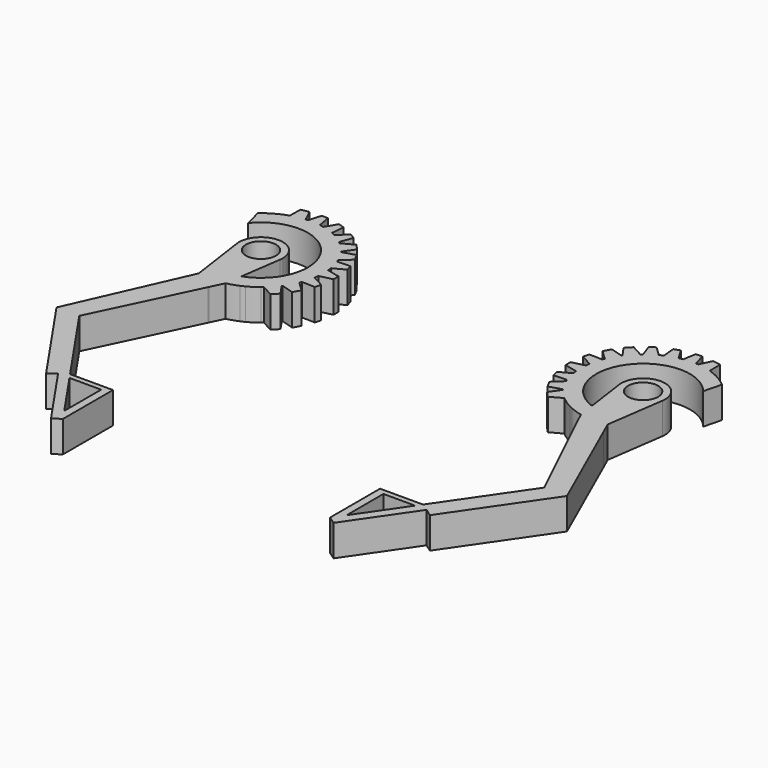
from build123d import *

# Parameters (mm, degrees)
F0_R     = 2.4
F1_DEPTH = 5
F2_DEPTH = 5


# Not quite as in the source:
# - a feature names something its author has since deleted; it is built from what else it names


with BuildPart() as f1:
    # F0 (on Top) → F1 (new body)
    with BuildSketch(Plane.XY):
        with BuildLine():
            Line((-28.0220931123, -7.0605402827), (-28.4076857165, -9.7674623873))
            ThreePointArc((-28.4076857165, -9.7674623873), (-27.4606084204, -9.510274656), (-26.5433011896, -9.1614933807))
            ThreePointArc((-26.5433011896, -9.1614933807), (-26.2465613416, -9.0258528435), (-25.9544044087, -8.8806040249))
            ThreePointArc((-25.9544044087, -8.8806040249), (-25.1052819595, -8.3867056795), (-24.3087141549, -7.811880278))
            ThreePointArc((-24.3087141549, -7.811880278), (-24.1632529957, -7.6933801849), (-24.0200406381, -7.572171928))
            ThreePointArc((-24.0200406381, -7.572171928), (-23.2137191877, -6.7937062036), (-22.4995744015, -5.9299004442))
            ThreePointArc((-22.4995744015, -5.9299004442), (-22.4615023659, -5.8778525229), (-22.4237667572, -5.8255601731))
            ThreePointArc((-22.4237667572, -5.8255601731), (-21.8229215363, -4.8794374612), (-21.3317236675, -3.8720210532))
            ThreePointArc((-21.3317236675, -3.8720210532), (-21.2607028173, -3.698362596), (-21.1929525017, -3.5234022701))
            ThreePointArc((-21.1929525017, -3.5234022701), (-20.8924140467, -2.588190451), (-20.685082074, -1.6280040303))
            ThreePointArc((-20.685082074, -1.6280040303), (-20.6372236959, -1.3052619222), (-20.5999195351, -0.981130325))
            ThreePointArc((-20.5999195351, -0.981130325), (-20.5516723096, 0), (-20.5999195351, 0.981130325))
            ThreePointArc((-20.5999195351, 0.981130325), (-20.6372236959, 1.3052619222), (-20.685082074, 1.6280040303))
            ThreePointArc((-20.685082074, 1.6280040303), (-20.8924140467, 2.588190451), (-21.1929525017, 3.5234022701))
            ThreePointArc((-21.1929525017, 3.5234022701), (-21.2607028173, 3.698362596), (-21.3317236675, 3.8720210532))
            ThreePointArc((-21.3317236675, 3.8720210532), (-21.8229215363, 4.8794374612), (-22.4237667572, 5.8255601731))
            ThreePointArc((-22.4237667572, 5.8255601731), (-22.4615023659, 5.8778525229), (-22.4995744015, 5.9299004442))
            ThreePointArc((-22.4995744015, 5.9299004442), (-23.2137191877, 6.7937062036), (-24.0200406381, 7.572171928))
            ThreePointArc((-24.0200406381, 7.572171928), (-24.1632529957, 7.6933801849), (-24.3087141549, 7.811880278))
            ThreePointArc((-24.3087141549, 7.811880278), (-25.1052819595, 8.3867056795), (-25.9544044087, 8.8806040249))
            ThreePointArc((-25.9544044087, 8.8806040249), (-26.2465613416, 9.0258528435), (-26.5433011896, 9.1614933807))
            ThreePointArc((-26.5433011896, 9.1614933807), (-27.4615023659, 9.510565163), (-28.4095219674, 9.7678652689))
            ThreePointArc((-28.4095219674, 9.7678652689), (-28.7293170547, 9.8325490756), (-29.0510520919, 9.8867658495))
            ThreePointArc((-29.0510520919, 9.8867658495), (-30.0283127472, 9.9862953475), (-31.0106235319, 9.989462637))
            ThreePointArc((-31.0106235319, 9.989462637), (-31.1979566888, 9.979093972), (-31.3850623458, 9.965212544))
            ThreePointArc((-31.3850623458, 9.965212544), (-32.4949607744, 9.8093644006), (-33.580448329, 9.5302946347))
            ThreePointArc((-33.580448329, 9.5302946347), (-33.6418422534, 9.510565163), (-33.7031076741, 9.4904401976))
            ThreePointArc((-33.7031076741, 9.4904401976), (-34.7453186457, 9.0781788046), (-35.7348505768, 8.5518806734))
            ThreePointArc((-35.7348505768, 8.5518806734), (-35.8943815316, 8.4531330387), (-36.0520317876, 8.3514097979))
            ThreePointArc((-36.0520317876, 8.3514097979), (-36.5923235865, 7.9693495438), (-37.1061642634, 7.5523926823))
            Line((-37.1061642634, 7.5523926823), (-36.3837682078, 4.7155760448))
            ThreePointArc((-36.3837682078, 4.7155760448), (-24.4364549725, 4.3421327617), (-28.0220931123, -7.0605402827))
        make_face()
        with BuildLine():
            ThreePointArc((-34.0166942863, -0.4935815043), (-30.5516723066, -3.5), (-27.0866503321, -0.4935814983))
            ThreePointArc((-27.0866503321, -0.4935814983), (-27.0604277664, -0.247409659), (-27.0516723096, 0))
            ThreePointArc((-27.0516723096, 0), (-30.7990819717, 3.491244543), (-34.0166942863, -0.4935815043))
        make_face()
        with Locations((-30.5516723096, 0)):
            Circle(F0_R, mode=Mode.SUBTRACT)
        with BuildLine():
            Line((-28.4086043831, -9.7693792448), (-28.4076857165, -9.7674623873))
            Line((-28.4076857165, -9.7674623873), (-28.0220931123, -7.0605402827))
            Line((-28.0220931123, -7.0605402827), (-27.0866503321, -0.4935814983))
            ThreePointArc((-27.0866503321, -0.4935814983), (-30.5516723066, -3.5), (-34.0166942863, -0.4935815043))
            Line((-34.0166942863, -0.4935815043), (-32.6956589028, -9.7674623873))
            Line((-32.6956589028, -9.7674623873), (-33.5248075263, -11.635811156))
            Line((-33.5248075263, -11.635811156), (-40.8083886817, -28.0481520771))
            Line((-40.8083886817, -28.0481520771), (-30.6916443131, -42.7764088872))
            Line((-30.6916443131, -42.7764088872), (-29.4552314726, -41.9271249018))
            Line((-29.4552314726, -41.9271249018), (-28.2188186321, -41.0778409164))
            Line((-28.2188186321, -41.0778409164), (-37.1688276447, -28.0481520771))
            Line((-37.1688276447, -28.0481520771), (-29.458068871, -11.9591548243))
            Line((-29.458068871, -11.9591548243), (-29.4044920171, -11.8473632511))
            Line((-29.4044920171, -11.8473632511), (-28.4086043831, -9.7693792448))
        make_face()
        Polygon((-21.3498832929, -41.0778409164), (-28.2188186321, -41.0778409164), (-29.4552314726, -41.9271249018), (-22.5862961334, -51.9271249018), (-21.3498832929, -51.0778409164), align=None)
        Polygon((-22.5791282712, -49.2882695816), (-27.635450954, -41.9271249018), (-22.5591333629, -41.9271249018), align=None, mode=Mode.SUBTRACT)
        with BuildLine():
            ThreePointArc((-20.5999195351, 0.981130325), (-20.5516723096, 0), (-20.5999195351, -0.981130325))
            Line((-20.5999195351, -0.981130325), (-18.5516723096, -0.5))
            Line((-18.5516723096, -0.5), (-18.5516723096, 0.5))
            Line((-18.5516723096, 0.5), (-20.5999195351, 0.981130325))
        make_face()
        with BuildLine():
            ThreePointArc((-20.685082074, -1.6280040303), (-20.8924140467, -2.588190451), (-21.1929525017, -3.5234022701))
            Line((-21.1929525017, -3.5234022701), (-19.0899719167, -3.5887914544))
            Line((-19.0899719167, -3.5887914544), (-18.8311528716, -2.6228656281))
            Line((-18.8311528716, -2.6228656281), (-20.685082074, -1.6280040303))
        make_face()
        with BuildLine():
            ThreePointArc((-21.3317236675, -3.8720210532), (-21.8229215363, -4.8794374612), (-22.4237667572, -5.8255601731))
            Line((-22.4237667572, -5.8255601731), (-20.4093674642, -6.4330127019))
            Line((-20.4093674642, -6.4330127019), (-19.8019921878, -5.309491614))
            Line((-19.8019921878, -5.309491614), (-21.3317236675, -3.8720210532))
        make_face()
        with BuildLine():
            ThreePointArc((-22.4237667572, 5.8255601731), (-21.8229215363, 4.8794374612), (-21.3317236675, 3.8720210532))
            Line((-21.3317236675, 3.8720210532), (-19.8019921878, 5.309491614))
            Line((-19.8019921878, 5.309491614), (-20.4093674642, 6.4330127019))
            Line((-20.4093674642, 6.4330127019), (-22.4237667572, 5.8255601731))
        make_face()
        with BuildLine():
            ThreePointArc((-21.1929525017, 3.5234022701), (-20.8924140467, 2.588190451), (-20.685082074, 1.6280040303))
            Line((-20.685082074, 1.6280040303), (-18.8311528716, 2.6228656281))
            Line((-18.8311528716, 2.6228656281), (-19.0899719167, 3.5887914544))
            Line((-19.0899719167, 3.5887914544), (-21.1929525017, 3.5234022701))
        make_face()
    extrude(amount=F1_DEPTH)

    # F0 (on Top) → F2 (join)
    with BuildSketch(Plane.XY):
        with BuildLine():
            ThreePointArc((-22.4995744015, -5.9299004442), (-23.2137191877, -6.7937062036), (-24.0200406381, -7.572171928))
            Line((-24.0200406381, -7.572171928), (-22.1802118701, -8.5828301877))
            Line((-22.1802118701, -8.5828301877), (-21.2993691007, -7.6579948636))
            Line((-21.2993691007, -7.6579948636), (-22.4995744015, -5.9299004442))
        make_face()
        with BuildLine():
            Line((-22.1802118701, 8.5828301877), (-24.0200406381, 7.572171928))
            ThreePointArc((-24.0200406381, 7.572171928), (-23.2137191877, 6.7937062036), (-22.4995744015, 5.9299004442))
            Line((-22.4995744015, 5.9299004442), (-21.2993691007, 7.6579948636))
            Line((-21.2993691007, 7.6579948636), (-22.1802118701, 8.5828301877))
        make_face()
        with BuildLine():
            Line((-24.4353391734, 10.3363663329), (-25.9544044087, 8.8806040249))
            ThreePointArc((-25.9544044087, 8.8806040249), (-25.1052819595, 8.3867056795), (-24.3087141549, 7.811880278))
            Line((-24.3087141549, 7.811880278), (-23.5966686055, 9.7917272978))
            Line((-23.5966686055, 9.7917272978), (-24.4353391734, 10.3363663329))
        make_face()
        with BuildLine():
            Line((-27.3189966353, 11.5671866927), (-28.4095219674, 9.7678652689))
            ThreePointArc((-28.4095219674, 9.7678652689), (-27.4615023659, 9.510565163), (-26.5433011896, 9.1614933807))
            Line((-26.5433011896, 9.1614933807), (-26.367940119, 11.2581696984))
            Line((-26.367940119, 11.2581696984), (-27.3189966353, 11.5671866927))
        make_face()
        with BuildLine():
            Line((-30.4229556021, 12.0097223952), (-31.0106235319, 9.989462637))
            ThreePointArc((-31.0106235319, 9.989462637), (-30.0283127472, 9.9862953475), (-29.0510520919, 9.8867658495))
            Line((-29.0510520919, 9.8867658495), (-29.4243260673, 11.9573864389))
            Line((-29.4243260673, 11.9573864389), (-30.4229556021, 12.0097223952))
        make_face()
        with BuildLine():
            Line((-33.5356863998, 11.6338153634), (-33.580448329, 9.5302946347))
            ThreePointArc((-33.580448329, 9.5302946347), (-32.4949607744, 9.8093644006), (-31.3850623458, 9.965212544))
            Line((-31.3850623458, 9.965212544), (-32.2794650656, 11.8642764682))
            Line((-32.2794650656, 11.8642764682), (-33.5356863998, 11.6338153634))
        make_face()
    extrude(amount=F2_DEPTH)


with BuildPart() as f3_1:
    # F3: instance of F1
    add(f1.part.mirror(Plane.YZ))


solid = Compound([f1.part, f3_1.part])
